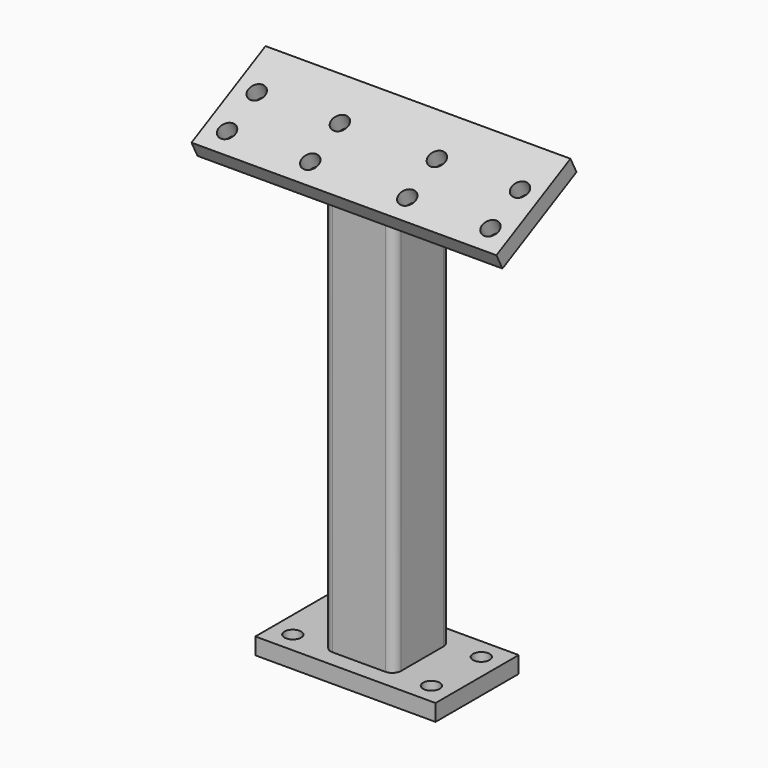
from build123d import *

# Parameters (mm, degrees)
F0_W      = 130
F0_H      = 75
F1_DEPTH  = 12
F3_DEPTH  = 319
F5_DEPTH  = 100
F6_W      = 220
F6_H      = 75
F7_DEPTH  = 12
F9_D      = 12
F9_DEPTH  = 12
F9_TIP    = 3.6051637142
F11_D     = 12
F11_DEPTH = 12
F11_TIP   = 3.6051637142


# Not quite as in the source:
# - a feature names something its author has since deleted; it is built from what else it names


with BuildPart() as f1:
    # F0 (on Top) → F1 (new body)
    with BuildSketch(Plane.XY):
        with Locations((65, -37.5)):
            Rectangle(F0_W, F0_H)
    extrude(amount=F1_DEPTH)

    # F2 (on face) → F3 (join)
    with BuildSketch(Plane.XY.offset(12)):
        with BuildLine():
            ThreePointArc((90.4, -18.45), (88.5401280605, -13.9598719395), (84.05, -12.1))
            Line((84.05, -12.1), (45.95, -12.1))
            ThreePointArc((45.95, -12.1), (41.4598719395, -13.9598719395), (39.6, -18.45))
            Line((39.6, -18.45), (39.6, -56.55))
            ThreePointArc((39.6, -56.55), (41.4598719395, -61.0401280605), (45.95, -62.9))
            Line((45.95, -62.9), (84.05, -62.9))
            ThreePointArc((84.05, -62.9), (88.5401280605, -61.0401280605), (90.4, -56.55))
            Line((90.4, -56.55), (90.4, -18.45))
        make_face()
        with BuildLine():
            Line((52.3, -18.45), (77.7, -18.45))
            ThreePointArc((77.7, -18.45), (82.1901280605, -20.3098719395), (84.05, -24.8))
            Line((84.05, -24.8), (84.05, -50.2))
            ThreePointArc((84.05, -50.2), (82.1901280605, -54.6901280605), (77.7, -56.55))
            Line((77.7, -56.55), (52.3, -56.55))
            ThreePointArc((52.3, -56.55), (47.8098719395, -54.6901280605), (45.95, -50.2))
            Line((45.95, -50.2), (45.95, -24.8))
            ThreePointArc((45.95, -24.8), (47.8098719395, -20.3098719395), (52.3, -18.45))
        make_face(mode=Mode.SUBTRACT)
    extrude(amount=F3_DEPTH)

    # F4 (on face) → F5 (cut)
    with BuildSketch(Plane.YZ.offset(90.4)):
        Polygon((-62.9, 305), (-12.1, 331), (-62.9, 331), align=None)
    extrude(amount=-F5_DEPTH, mode=Mode.SUBTRACT)

    # F6 (on face) → F7 (join)
    with BuildSketch(Plane(origin=(0, -136.7557973863, 267.1997887393), x_dir=(1, 0, 0), z_dir=(0, -0.4556049895, 0.8901820564))):
        with Locations((65, 111.5005595453)):
            Rectangle(F6_W, F6_H)
        with BuildLine():
            Line((90.4, 132.9006763674), (90.4, 90.1004427232))
            add(Edge.make_bspline(
                [(90.4, 90.1004427232), (90.4, 82.9670704491), (84.05, 82.9670704491)],
                knots=[4.7123889804, 4.7123889804, 4.7123889804, 6.2831853072, 6.2831853072, 6.2831853072], degree=2, weights=[1, 0.7071067812, 1]))
            Line((84.05, 82.9670704491), (45.95, 82.9670704491))
            add(Edge.make_bspline(
                [(45.95, 82.9670704491), (39.6, 82.9670704491), (39.6, 90.1004427232)],
                knots=[0, 0, 0, 1.5707963268, 1.5707963268, 1.5707963268], degree=2, weights=[1, 0.7071067812, 1]))
            Line((39.6, 90.1004427232), (39.6, 132.9006763674))
            add(Edge.make_bspline(
                [(39.6, 132.9006763674), (39.6, 140.0340486414), (45.95, 140.0340486414)],
                knots=[1.5707963268, 1.5707963268, 1.5707963268, 3.1415926536, 3.1415926536, 3.1415926536], degree=2, weights=[1, 0.7071067812, 1]))
            Line((45.95, 140.0340486414), (84.05, 140.0340486414))
            add(Edge.make_bspline(
                [(84.05, 140.0340486414), (90.4, 140.0340486414), (90.4, 132.9006763674)],
                knots=[3.1415926536, 3.1415926536, 3.1415926536, 4.7123889804, 4.7123889804, 4.7123889804], degree=2, weights=[1, 0.7071067812, 1]))
        make_face(mode=Mode.SUBTRACT)
        with BuildLine():
            add(Edge.make_bspline(
                [(90.4, 90.1004427232), (90.4, 82.9670704491), (84.05, 82.9670704491)],
                knots=[4.7123889804, 4.7123889804, 4.7123889804, 6.2831853072, 6.2831853072, 6.2831853072], degree=2, weights=[1, 0.7071067812, 1]))
            Line((90.4, 90.1004427232), (90.4, 132.9006763674))
            add(Edge.make_bspline(
                [(84.05, 140.0340486414), (90.4, 140.0340486414), (90.4, 132.9006763674)],
                knots=[3.1415926536, 3.1415926536, 3.1415926536, 4.7123889804, 4.7123889804, 4.7123889804], degree=2, weights=[1, 0.7071067812, 1]))
            Line((84.05, 140.0340486414), (45.95, 140.0340486414))
            add(Edge.make_bspline(
                [(39.6, 132.9006763674), (39.6, 140.0340486414), (45.95, 140.0340486414)],
                knots=[1.5707963268, 1.5707963268, 1.5707963268, 3.1415926536, 3.1415926536, 3.1415926536], degree=2, weights=[1, 0.7071067812, 1]))
            Line((39.6, 132.9006763674), (39.6, 90.1004427232))
            add(Edge.make_bspline(
                [(45.95, 82.9670704491), (39.6, 82.9670704491), (39.6, 90.1004427232)],
                knots=[0, 0, 0, 1.5707963268, 1.5707963268, 1.5707963268], degree=2, weights=[1, 0.7071067812, 1]))
            Line((45.95, 82.9670704491), (84.05, 82.9670704491))
        make_face()
        with BuildLine():
            Line((52.3, 132.9006763674), (77.7, 132.9006763674))
            add(Edge.make_bspline(
                [(77.7, 132.9006763674), (84.05, 132.9006763674), (84.05, 125.7673040934)],
                knots=[3.1415926536, 3.1415926536, 3.1415926536, 4.7123889804, 4.7123889804, 4.7123889804], degree=2, weights=[1, 0.7071067812, 1]))
            Line((84.05, 125.7673040934), (84.05, 97.2338149972))
            add(Edge.make_bspline(
                [(84.05, 97.2338149972), (84.05, 90.1004427232), (77.7, 90.1004427232)],
                knots=[4.7123889804, 4.7123889804, 4.7123889804, 6.2831853072, 6.2831853072, 6.2831853072], degree=2, weights=[1, 0.7071067812, 1]))
            Line((77.7, 90.1004427232), (52.3, 90.1004427232))
            add(Edge.make_bspline(
                [(52.3, 90.1004427232), (45.95, 90.1004427232), (45.95, 97.2338149972)],
                knots=[0, 0, 0, 1.5707963268, 1.5707963268, 1.5707963268], degree=2, weights=[1, 0.7071067812, 1]))
            Line((45.95, 97.2338149972), (45.95, 125.7673040934))
            add(Edge.make_bspline(
                [(45.95, 125.7673040934), (45.95, 132.9006763674), (52.3, 132.9006763674)],
                knots=[1.5707963268, 1.5707963268, 1.5707963268, 3.1415926536, 3.1415926536, 3.1415926536], degree=2, weights=[1, 0.7071067812, 1]))
        make_face(mode=Mode.SUBTRACT)
        with BuildLine():
            add(Edge.make_bspline(
                [(77.7, 132.9006763674), (84.05, 132.9006763674), (84.05, 125.7673040934)],
                knots=[3.1415926536, 3.1415926536, 3.1415926536, 4.7123889804, 4.7123889804, 4.7123889804], degree=2, weights=[1, 0.7071067812, 1]))
            Line((77.7, 132.9006763674), (52.3, 132.9006763674))
            add(Edge.make_bspline(
                [(45.95, 125.7673040934), (45.95, 132.9006763674), (52.3, 132.9006763674)],
                knots=[1.5707963268, 1.5707963268, 1.5707963268, 3.1415926536, 3.1415926536, 3.1415926536], degree=2, weights=[1, 0.7071067812, 1]))
            Line((45.95, 125.7673040934), (45.95, 97.2338149972))
            add(Edge.make_bspline(
                [(52.3, 90.1004427232), (45.95, 90.1004427232), (45.95, 97.2338149972)],
                knots=[0, 0, 0, 1.5707963268, 1.5707963268, 1.5707963268], degree=2, weights=[1, 0.7071067812, 1]))
            Line((52.3, 90.1004427232), (77.7, 90.1004427232))
            add(Edge.make_bspline(
                [(84.05, 97.2338149972), (84.05, 90.1004427232), (77.7, 90.1004427232)],
                knots=[4.7123889804, 4.7123889804, 4.7123889804, 6.2831853072, 6.2831853072, 6.2831853072], degree=2, weights=[1, 0.7071067812, 1]))
            Line((84.05, 97.2338149972), (84.05, 125.7673040934))
        make_face()
    extrude(amount=F7_DEPTH)

    # F9
    with Locations(Plane(origin=(0, -142.2230572602, 277.8819734162), x_dir=(1, 0, 0), z_dir=(0, -0.4556049895, 0.8901820564))):
        with Locations((-30, 89.0005595453), (100, 89.0005595453), (160, 89.0005595453), (160, 119.0005595453), (100, 119.0005595453), (30, 119.0005595453), (-30, 119.0005595453), (30, 89.0005595453)):
            Hole(F9_D / 2, depth=F9_DEPTH)
            with Locations((0, 0, -(F9_DEPTH + F9_TIP / 2))):  # 118° drill point
                Cone(0, F9_D / 2, F9_TIP, mode=Mode.SUBTRACT)

    # F11 (one way)
    with BuildSketch(Plane.XY.offset(12)):
        with Locations((15, -15), (15, -60), (115, -60), (115, -15)):
            Circle(F11_D / 2)
    extrude(amount=-F11_DEPTH, mode=Mode.SUBTRACT)
    with Locations(Plane.XY.offset(12)):
        with Locations((15, -15), (15, -60), (115, -60), (115, -15)):
            with Locations((0, 0, -(F11_DEPTH + F11_TIP / 2))):  # 118° drill point
                Cone(0, F11_D / 2, F11_TIP, mode=Mode.SUBTRACT)


solid = f1.part
